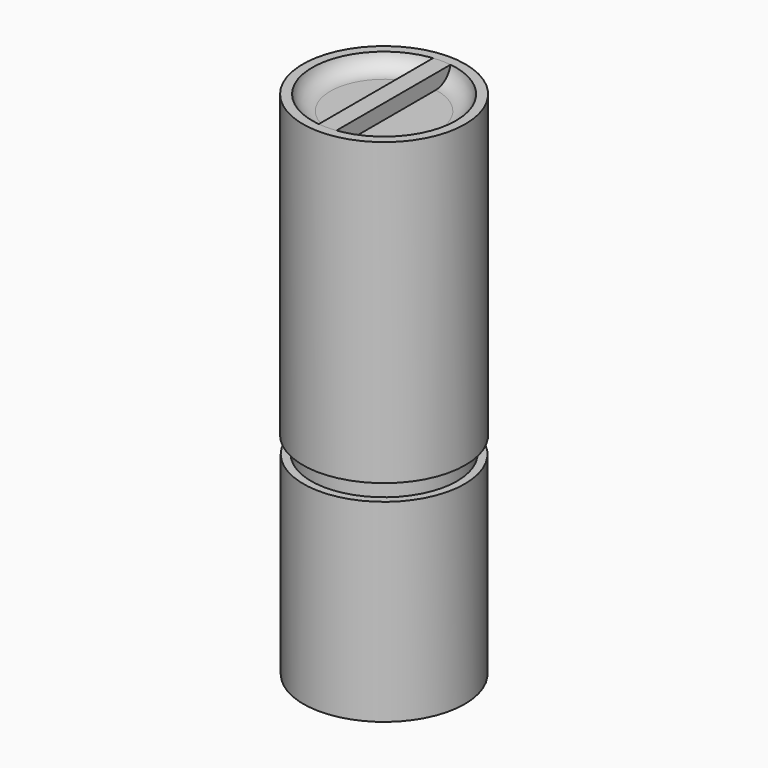
from build123d import *

# Parameters (mm, degrees)
F0_R      = 33.1221613945
F1_DEPTH  = 79.502
F2_R      = 29.9522541519
F3_DEPTH  = 6.858
F4_R      = 33.3382653076
F4_R_2    = 29.9522541519
F5_DEPTH  = 123.19
F6_R      = 29.5084253816
F7_DEPTH  = 6.096
F10_DEPTH = 25.4


# Not quite as in the source:
# - a fillet or chamfer that OpenCascade refuses, or shapes differently, is made with other operations: its cross-section is extruded or revolved along the edge and cut away or added


with BuildPart() as f1:
    # F0 (on Top) → F1 (new body)
    with BuildSketch(Plane.XY):
        with Locations((-20.5001533031, 21.8376107514)):
            Circle(F0_R)
    extrude(amount=F1_DEPTH)

    # F2 (on face) → F3 (join)
    with BuildSketch(Plane.XY.offset(79.502)):
        with Locations((-20.5001533031, 21.8376107514)):
            Circle(F2_R)
    extrude(amount=F3_DEPTH)

    # F4 (on face) → F5 (join)
    with BuildSketch(Plane.XY.offset(86.36)):
        with Locations((-20.5001533031, 21.8376107514)):
            Circle(F4_R)
        with Locations((-20.5001533031, 21.8376107514)):
            Circle(F4_R_2, mode=Mode.SUBTRACT)
        with Locations((-20.5001533031, 21.8376107514)):
            Circle(F4_R_2)
    extrude(amount=F5_DEPTH)

    # F6 (on face) → F7 (cut)
    with BuildSketch(Plane.XY.offset(209.55)):
        with Locations((-20.5001533031, 21.8376107514)):
            Circle(F6_R)
    extrude(amount=-F7_DEPTH, mode=Mode.SUBTRACT)

    # F8: fillet of radius 7.62 on 1 edges, made by hand

    # F8_s1 → F8_t2 (revolve)
    with BuildSketch(Plane.XZ.offset(-21.8376107514)):
        with BuildLine():
            ThreePointArc((9.0082720785, 209.55), (6.3615384966, 205.1715733804), (1.5422273425, 203.454))
            Line((1.5422273425, 203.454), (9.0082720785, 203.454))
            Line((9.0082720785, 203.454), (9.0082720785, 209.55))
        make_face()
    revolve(axis=Axis((-20.5001533031, 21.8376107514, 203.454), (0, 0, 1)))


with BuildPart() as f10:
    # F9 (on face) → F10 (new body)
    with BuildSketch(Plane.XY.offset(209.55)):
        with BuildLine():
            ThreePointArc((-16.6392866522, 51.0923689491), (-20.2408198189, 51.3448965406), (-23.8462351263, 51.1557093415))
            Line((-23.8462351263, 51.1557093415), (-23.8462351263, -7.4804878387))
            ThreePointArc((-23.8462351263, -7.4804878387), (-20.2408198189, -7.6696750378), (-16.6392866522, -7.4171474463))
            Line((-16.6392866522, -7.4171474463), (-16.6392866522, 51.0923689491))
        make_face()
    extrude(amount=-F10_DEPTH)


solid = Compound([f1.part, f10.part])
